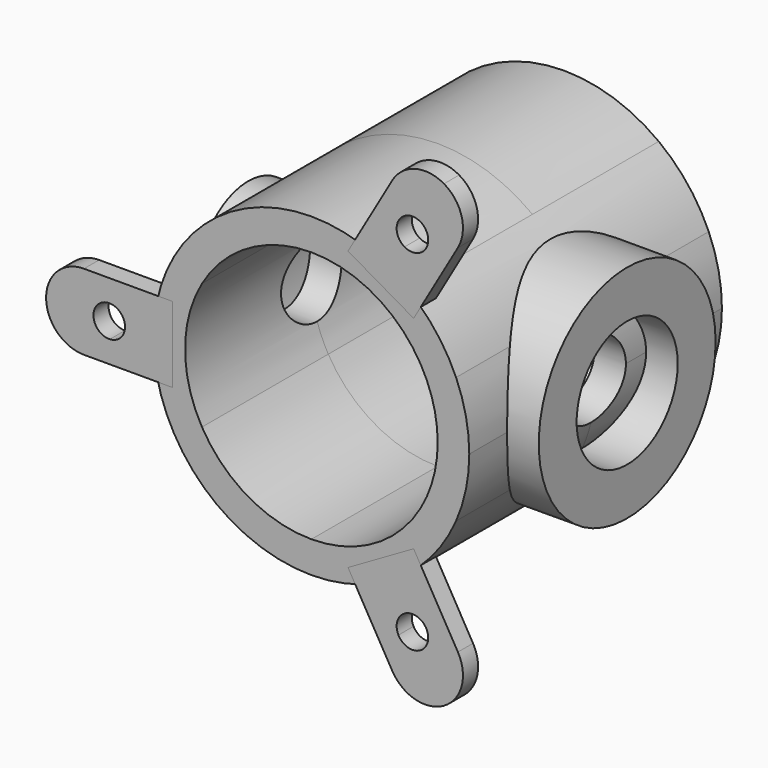
from build123d import *

# Parameters (mm, degrees)
F1_DEPTH      = 125
F3_R          = 87.5
F3_R_2        = 50
F3_R_3        = 30
F5_DEPTH      = 275
F8_END_RADIUS = 125
F7_R          = 50
F8_REACH      = 441.4223563373
F11_DEPTH     = 15
F12_R         = 29.99999
F13_COUNT     = 3


# Not quite as in the source:
# - a fillet or chamfer is up to 0.001 mm smaller than in the source, because OpenCascade refuses the exact size


with BuildPart() as f1:
    # F0 (on Front) → F1 (new body, symmetric)
    with BuildSketch(Plane.XZ):
        with BuildLine():
            ThreePointArc((-86.6025403784, 50), (-50.0000000221, 86.6025403657), (-5.1e-08, 100))
            Line((-5.1e-08, 100), (-75, 100))
            ThreePointArc((-75, 100), (-98.0237966721, 77.5650390703), (-114.5643923739, 50))
            Line((-114.5643923739, 50), (-86.6025403784, 50))
        make_face()
        with BuildLine():
            ThreePointArc((-5.1e-08, 100), (49.9999999779, 86.6025403912), (86.6025403784, 50))
            Line((86.6025403784, 50), (114.5643923739, 50))
            ThreePointArc((114.5643923739, 50), (98.0237966721, 77.5650390703), (75, 100))
            Line((75, 100), (-5.1e-08, 100))
        make_face()
        with BuildLine():
            Line((75, -100), (1.33e-07, -100))
            Line((1.33e-07, -100), (-75, -100))
            ThreePointArc((-75, -100), (0, -125), (75, -100))
        make_face()
        with BuildLine():
            ThreePointArc((-86.6025403784, -50), (-100, 0), (-86.6025403784, 50))
            Line((-86.6025403784, 50), (-114.5643923739, 50))
            ThreePointArc((-114.5643923739, 50), (-125, 0), (-114.5643923739, -50))
            Line((-114.5643923739, -50), (-86.6025403784, -50))
        make_face()
        with BuildLine():
            Line((-75, -100), (1.33e-07, -100))
            ThreePointArc((1.33e-07, -100), (-49.9999999424, -86.6025404117), (-86.6025403784, -50))
            Line((-86.6025403784, -50), (-114.5643923739, -50))
            ThreePointArc((-114.5643923739, -50), (-98.0237966721, -77.5650390703), (-75, -100))
        make_face()
        with BuildLine():
            Line((114.5643923739, -50), (86.6025403784, -50))
            ThreePointArc((86.6025403784, -50), (50.0000000576, -86.6025403452), (1.33e-07, -100))
            Line((1.33e-07, -100), (75, -100))
            ThreePointArc((75, -100), (98.0237966721, -77.5650390703), (114.5643923739, -50))
        make_face()
        with BuildLine():
            ThreePointArc((86.6025403784, 50), (96.5925826289, 25.8819045103), (100, 0))
            ThreePointArc((100, 0), (96.5925826289, -25.8819045103), (86.6025403784, -50))
            Line((86.6025403784, -50), (114.5643923739, -50))
            ThreePointArc((114.5643923739, -50), (122.3632891163, -25.5387054612), (125, 0))
            ThreePointArc((125, 0), (122.3632891163, 25.5387054612), (114.5643923739, 50))
            Line((114.5643923739, 50), (86.6025403784, 50))
        make_face()
        with BuildLine():
            Line((-75, 100), (-5.1e-08, 100))
            Line((-5.1e-08, 100), (75, 100))
            ThreePointArc((75, 100), (0, 125), (-75, 100))
        make_face()
    extrude(amount=F1_DEPTH, both=True)

    # F3 (on offset) → F4 (join, up to the next surface of F1)
    with BuildSketch(Plane.YZ.offset(150)):
        Circle(F3_R)
        Circle(F3_R_2, mode=Mode.SUBTRACT)
    extrude(until=Until.NEXT, dir=(-1, 0, 0))

    # F3 (on offset) → F5 (cut)
    with BuildSketch(Plane.YZ.offset(150)):
        Circle(F3_R_3)
    extrude(amount=-F5_DEPTH, mode=Mode.SUBTRACT)

    f8_end = (Plane(origin=(0, 0, 0), x_dir=(0, 0, -1), z_dir=(0, -1, 0)) * Cylinder(F8_END_RADIUS, 1778.6683567252, mode=Mode.PRIVATE)).faces().sort_by_distance((-75, 0, -100))[0]
    # F7 (on offset) → F8 (join, up to the whole of a round face its end follows)
    with BuildSketch(Plane.YZ.offset(-150)):
        Circle(F7_R)
    f8_long = extrude(amount=F8_REACH, mode=Mode.PRIVATE)
    add(split(f8_long, bisect_by=f8_end, keep=Keep.ALL, mode=Mode.PRIVATE).solids().sort_by_distance((-150, 0, 0))[0])


with BuildPart() as f11:
    # F10 (on offset) → F11 (new body)
    with BuildSketch(Plane.XZ.offset(125)):
        with BuildLine():
            ThreePointArc((-159.51171875, 12.4904596161), (-158.5788772539, 21.2776805336), (-157.162336455, 30))
            Line((-157.162336455, 30), (-210, 30))
            Line((-210, 30), (-210, -30))
            Line((-210, -30), (-157.162336455, -30))
            ThreePointArc((-157.162336455, -30), (-158.5788772539, -21.2776805336), (-159.51171875, -12.4904596161))
            ThreePointArc((-159.51171875, -12.4904596161), (-172.5, 0), (-159.51171875, 12.4904596161))
        make_face()
        with BuildLine():
            Line((-110, 30), (-157.162336455, 30))
            ThreePointArc((-157.162336455, 30), (-158.5788772539, 21.2776805336), (-159.51171875, 12.4904596161))
            ThreePointArc((-159.51171875, 12.4904596161), (-150.9901854729, 8.6644816456), (-147.5, 0))
            ThreePointArc((-147.5, 0), (-150.9901854729, -8.6644816456), (-159.51171875, -12.4904596161))
            ThreePointArc((-159.51171875, -12.4904596161), (-158.5788772539, -21.2776805336), (-157.162336455, -30))
            Line((-157.162336455, -30), (-110, -30))
            Line((-110, -30), (-110, 30))
        make_face()
    extrude(amount=-F11_DEPTH)

    # F12 (radius 30 in the source; OpenCascade refuses exactly that, so slightly less here)
    f12_edges = [f11.edges().sort_by_distance(p)[0] for p in [
        (-210, -117.5, -30),
        (-210, -117.5, 30),
    ]]
    fillet(f12_edges, radius=F12_R)


with BuildPart() as f13_1:
    # F13: instance of F11
    add(f11.part.rotate(Axis((0, -125, 0), (0, -1, 0)), 1 * 360 / F13_COUNT))


with BuildPart() as f13_2:
    # F13: instance of F11
    add(f11.part.rotate(Axis((0, -125, 0), (0, -1, 0)), 2 * 360 / F13_COUNT))


solid = Compound([f1.part, f11.part, f13_1.part, f13_2.part])
